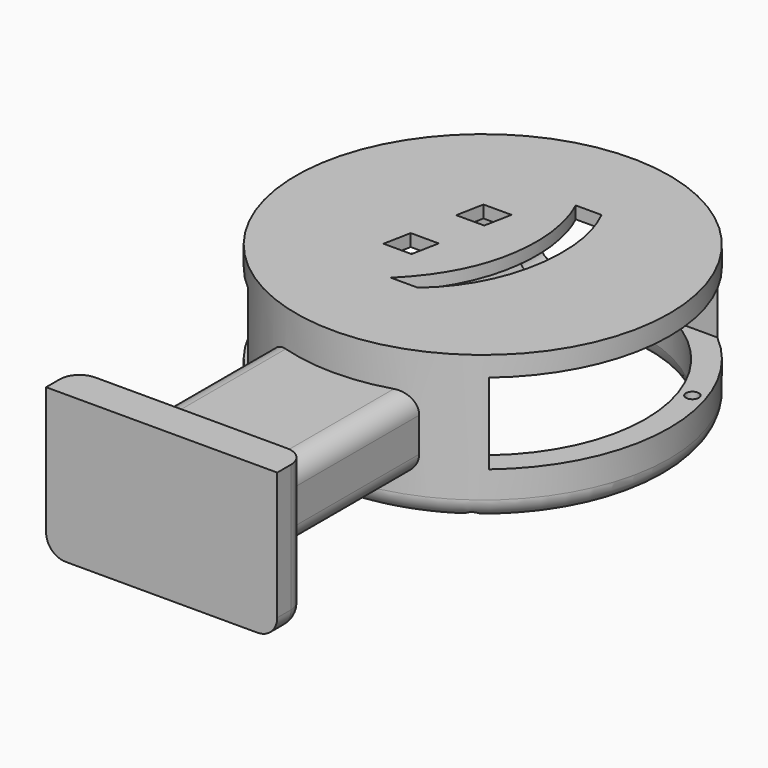
from build123d import *

# Parameters (mm, degrees)
F0_R           = 48.2681102906
F0_R_2         = 42.06875
F1_DEPTH       = 38.1
F2_R           = 46.0375
F3_DEPTH       = 3.175
F5_DEPTH       = 95.758
F7_W           = 38.1
F7_H           = 19.05
F8_DEPTH       = 50.8
F9_W           = 59.7543008626
F9_H           = 38.1
F10_DEPTH      = 9.525
F11_R          = 5.08
F12_R          = 1.6712655212
F13_DEPTH      = 12.7
F14_TEXT_SIZE  = 51.4914307536
F15_DEPTH      = 81.788
F16_W          = 73.8427117467
F16_H          = 20.8774539718
F17_DEPTH      = 108.712
F17_DEPTH_BACK = 64.008


# Not quite as in the source:
# - a fillet or chamfer that OpenCascade refuses, or shapes differently, is made with other operations: its cross-section is extruded or revolved along the edge and cut away or added
# - Text() gives the source's letters only with a copy of the font that has no kerning and outlines rounded to 1/6400 em; it was checked with that copy


with BuildPart() as f1:
    # F0 (on Top) → F1 (new body)
    with BuildSketch(Plane.XY):
        Circle(F0_R)
        Circle(F0_R_2, mode=Mode.SUBTRACT)
    extrude(amount=F1_DEPTH)

    # F2 (on face) → F3 (join)
    with BuildSketch(Plane.XY.offset(38.1)):
        Circle(F2_R)
    extrude(amount=-F3_DEPTH)

    # F4 (on Front) → F5 (cut)
    with BuildSketch(Plane.XZ):
        with BuildLine():
            Line((16.7659605317, 28.234812431), (-16.7659605317, 28.234812431))
            ThreePointArc((-16.7659605317, 28.234812431), (-19.011024562, 27.3048764613), (-19.9409605317, 25.059812431))
            Line((-19.9409605317, 25.059812431), (-19.9409605317, 13.040187569))
            ThreePointArc((-19.9409605317, 13.040187569), (-19.011024562, 10.7951235387), (-16.7659605317, 9.865187569))
            Line((-16.7659605317, 9.865187569), (0, 9.865187569))
            Line((0, 9.865187569), (16.7659605317, 9.865187569))
            ThreePointArc((16.7659605317, 9.865187569), (19.011024562, 10.7951235387), (19.9409605317, 13.040187569))
            Line((19.9409605317, 13.040187569), (19.9409605317, 25.059812431))
            ThreePointArc((19.9409605317, 25.059812431), (19.011024562, 27.3048764613), (16.7659605317, 28.234812431))
        make_face()
    extrude(amount=-F5_DEPTH, mode=Mode.SUBTRACT)

    # F7 (on offset) → F8 (join)
    with BuildSketch(Plane.XZ.offset(43.434)):
        with Locations((0, 19.05)):
            Rectangle(F7_W, F7_H)
    extrude(amount=F8_DEPTH)

    # F9 (on face) → F10 (join)
    with BuildSketch(Plane.XZ.offset(94.234)):
        with Locations((0, 19.05)):
            Rectangle(F9_W, F9_H)
    extrude(amount=F10_DEPTH)

    # F11
    f11_edges = [f1.edges().sort_by_distance(p)[0] for p in [
        (-29.87715, -98.9965, 0),
        (-29.87715, -94.234, 19.05),
        (-19.05, -69.291918, 9.525),
        (-19.05, -69.291918, 28.575),
        (19.05, -69.291918, 28.575),
        (19.05, -69.291918, 9.525),
        (29.87715, -94.234, 19.05),
        (0, -94.234, 0),
        (29.87715, -98.9965, 0),
    ]]
    fillet(f11_edges, radius=F11_R)

    # F12 (on Top) → F13 (cut)
    with BuildSketch(Plane.XY):
        with BuildLine():
            ThreePointArc((1.6712655212, 45.2193766832), (1.1817631832, 46.4011398664), (0, 46.8906422044))
            Line((0, 46.8906422044), (0, 43.548111162))
            ThreePointArc((0, 43.548111162), (1.1817631832, 44.0376135), (1.6712655212, 45.2193766832))
        make_face()
        with BuildLine():
            Line((0, 43.548111162), (0, 46.8906422044))
            ThreePointArc((0, 46.8906422044), (-1.6712655212, 45.2193766832), (0, 43.548111162))
        make_face()
        with Locations((-43.0061828574, 13.9735558702)):
            Circle(F12_R)
        with Locations((-26.5792827323, -36.5832442118)):
            Circle(F12_R)
        with Locations((26.5792827323, -36.5832442118)):
            Circle(F12_R)
        with Locations((43.0061828574, 13.9735558702)):
            Circle(F12_R)
    extrude(amount=F13_DEPTH, mode=Mode.SUBTRACT)

    # F14 (on face) → F15 (cut)
    with BuildSketch(Plane.XY.offset(38.1)):
        with Locations((-18.1079478934, -12.2418429237)):
            Text(':)', F14_TEXT_SIZE, font='Arimo', font_style=FontStyle.BOLDITALIC, text_align=(TextAlign.LEFT, TextAlign.BOTTOM))
    extrude(amount=-F15_DEPTH, mode=Mode.SUBTRACT)

    # F16 (on Right) → F17 (cut, two sides)
    with BuildSketch(Plane.YZ) as f17_sk:
        with Locations((0, 22.4966847957)):
            Rectangle(F16_W, F16_H)
    extrude(amount=-F17_DEPTH, mode=Mode.SUBTRACT)
    extrude(f17_sk.sketch, amount=F17_DEPTH_BACK, mode=Mode.SUBTRACT)

    # F18: fillet of radius 5.08 on 1 edges, made by hand

    # F18_s1 → F18_t2 (revolve, cut)
    with BuildSketch(Plane.XZ):
        with BuildLine():
            ThreePointArc((48.2681102906, 5.08), (46.780212739, 1.4878975516), (43.1881102906, 0))
            Line((43.1881102906, 0), (48.2681102906, 0))
            Line((48.2681102906, 0), (48.2681102906, 5.08))
        make_face()
    revolve(axis=Axis((0, 0, 0), (0, 0, 1)), mode=Mode.SUBTRACT)

    # F19: fillet of radius 5.08 on 1 edges, made by hand

    # F19_s1 → F19_t2 (revolve, cut)
    with BuildSketch(Plane.XZ):
        with BuildLine():
            ThreePointArc((42.06875, 3.181152793), (42.3567540837, 1.4949810526), (43.1881102906, 0))
            Line((43.1881102906, 0), (42.06875, 0))
            Line((42.06875, 0), (42.06875, 3.181152793))
        make_face()
    revolve(axis=Axis((0, 0, 0), (0, 0, 1)), mode=Mode.SUBTRACT)


solid = f1.part
